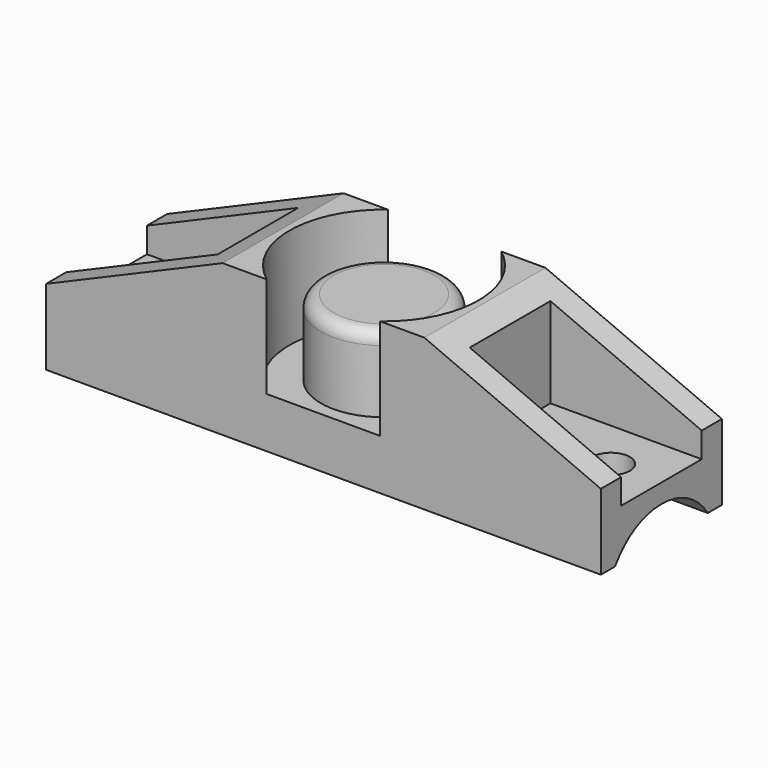
from build123d import *

# Parameters (mm, degrees)
F0_W         = 69.85
F0_H         = 19.05
F1_DEPTH     = 19.05
F2_R         = 11.90625
F3_DEPTH     = 12.7
F4_R         = 7.9375
F5_DEPTH     = 9.525
F6_W         = 38.1
F6_H         = 12.7
F7_DEPTH     = 12.7
F8_R         = 2.38125
F9_DEPTH     = 25.4
F10_R        = 8.6959968999
F11_DEPTH    = 69.851
F12_R        = 1.5875
F13_C1_SIZE2 = 9.525
F13_C1_SIZE  = 22.225
F13_C2_SIZE2 = 22.225
F13_C2_SIZE  = 9.525


# Not quite as in the source:
# - two fillets or chamfers of one size are made in one step


with BuildPart() as f1:
    # F0 (on Top) → F1 (new body)
    with BuildSketch(Plane.XY):
        with Locations((34.925, 9.525)):
            Rectangle(F0_W, F0_H)
    extrude(amount=F1_DEPTH)

    # F2 (on face) → F3 (cut)
    with BuildSketch(Plane.XY.offset(19.05)):
        with Locations((34.925, 9.525)):
            Circle(F2_R)
    extrude(amount=-F3_DEPTH, mode=Mode.SUBTRACT)

    # F4 (on face) → F5 (join)
    with BuildSketch(Plane.XY.offset(6.35)):
        with Locations((34.925, 9.525)):
            Circle(F4_R)
    extrude(amount=F5_DEPTH)

    # F6 (on face) → F7 (cut)
    with BuildSketch(Plane.XY.offset(19.05)):
        with Locations((69.85, 9.525)):
            Rectangle(F6_W, F6_H)
        with Locations((0, 9.525)):
            Rectangle(F6_W, F6_H)
    extrude(amount=-F7_DEPTH, mode=Mode.SUBTRACT)

    # F8 (on face) → F9 (cut)
    with BuildSketch(Plane.XY.offset(6.35)):
        with Locations((63.5, 9.525)):
            Circle(F8_R)
        with Locations((6.35, 9.5145329833)):
            Circle(F8_R)
    extrude(amount=-F9_DEPTH, mode=Mode.SUBTRACT)

    # F10 (on face) → F11 (cut, through all)
    with BuildSketch(Plane.YZ.offset(69.85)):
        with Locations((9.525, -4.7272468999)):
            Circle(F10_R)
    extrude(amount=-F11_DEPTH, mode=Mode.SUBTRACT)

    # F12
    f12_edges = [f1.edges().sort_by_distance(p)[0] for p in [
        (26.9875, 9.525, 15.875),
    ]]
    fillet(f12_edges, radius=F12_R)

    # F13: chamfer of 9.525 x 22.225 on 4 edges, made by hand

    # F13_c1
    f13_c1_edges = [f1.edges().sort_by_distance(p)[0] for p in [
        (69.85, 17.4625, 19.05),
    ]]
    f13_c1_side = f1.faces().sort_by_distance((69.6595, 17.4625, 19.05))[0]
    chamfer(f13_c1_edges, length=F13_C1_SIZE, length2=F13_C1_SIZE2, reference=f13_c1_side)

    # F13_c2
    f13_c2_edges = [f1.edges().sort_by_distance(p)[0] for p in [
        (0, 1.5875, 19.05),
    ]]
    f13_c2_side = f1.faces().sort_by_distance((0, 1.5875, 18.8595))[0]
    chamfer(f13_c2_edges, length=F13_C2_SIZE, length2=F13_C2_SIZE2, reference=f13_c2_side)


solid = f1.part
